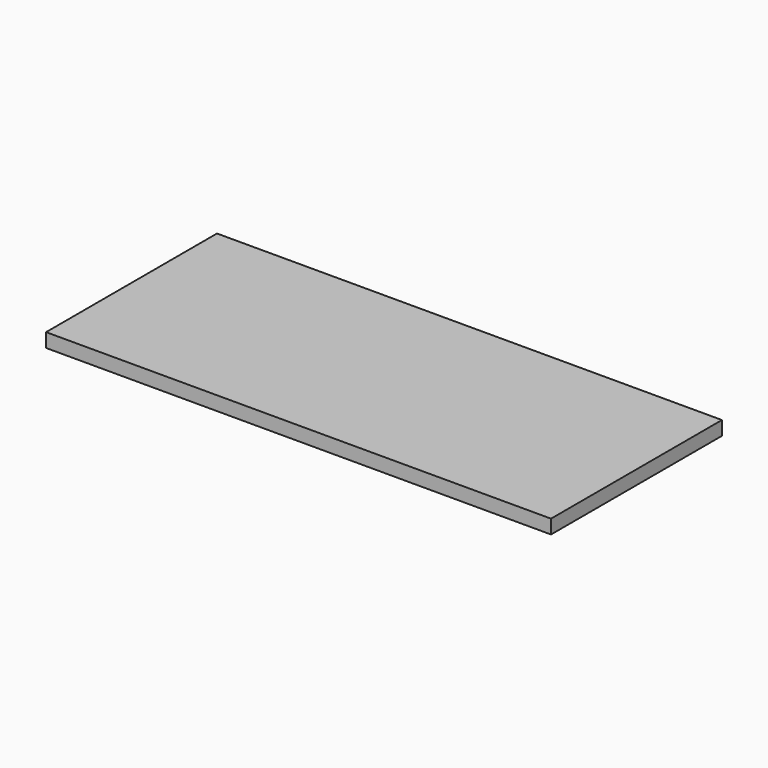
from build123d import *

# Parameters (mm, degrees)
F0_W     = 660.4
F0_H     = 279.4
F1_DEPTH = 18.25625


# Not quite as in the source:
# - a length typed as a fraction of an inch, garbled in the dataset ("3 / 203.2 mm" for 3/8 in), is restored


with BuildPart() as f1:
    # F0 (on Top) → F1 (new body)
    with BuildSketch(Plane.XY):
        with Locations((29.9875289202, 6.2856816543)):
            Rectangle(F0_W, F0_H)
    extrude(amount=F1_DEPTH)


solid = f1.part
